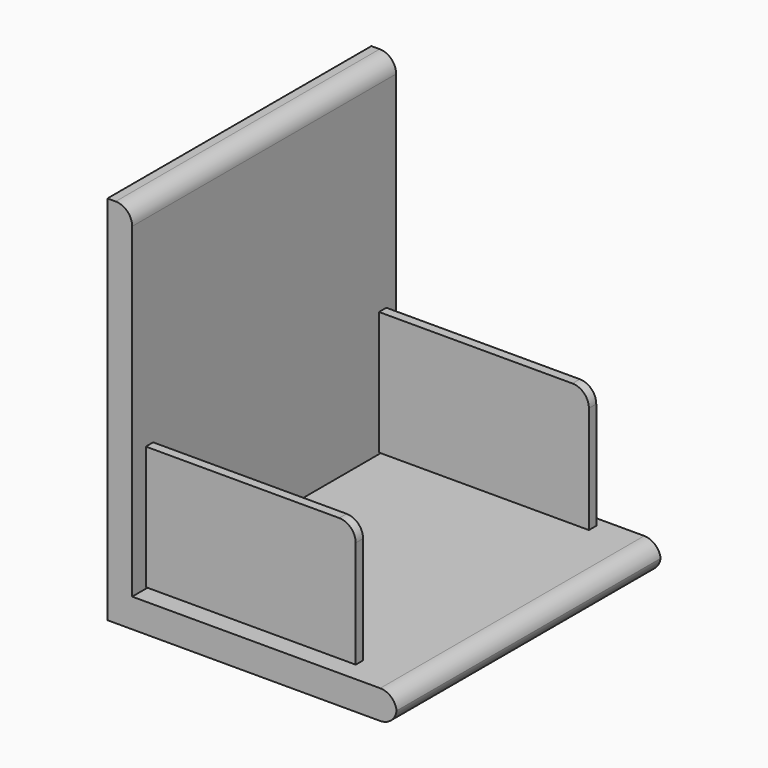
from build123d import *

# Parameters (mm, degrees)
F1_DEPTH      = 50.8
F2_W          = 64.6359566599
F2_H          = 2.8338059783
F3_DEPTH      = 38.1
F2_H_2        = 2.8299428523
F4_T1_DEPTH   = 127
F4_2_T1_DEPTH = 28.2338059783
F4_3_T1_DEPTH = 28.2299428523


# Not quite as in the source:
# - a fillet or chamfer that OpenCascade refuses, or shapes differently, is made with other operations: its cross-section is extruded or revolved along the edge and cut away or added


with BuildPart() as f1:
    # F0 (on Front) → F1 (new body, symmetric)
    with BuildSketch(Plane.XZ):
        Polygon((-46.0972779441, 66.8356441736), (-53.7172779441, 66.8356441736), (-53.7172779441, -47.4876239896), (-46.1948015571, -47.4876239896), (35.3699997067, -47.4876239896), (35.3699997067, -38.6183932424), (-46.0972779441, -38.6183932424), align=None)
    extrude(amount=F1_DEPTH, both=True)

    # F4: fillet of radius 5.08 on 3 edges, made by hand

    # F4_s2 → F4_t1 (cut)
    with BuildSketch(Plane.XZ.offset(-63.5)):
        with BuildLine():
            ThreePointArc((30.2899997067, -38.6183932424), (33.8821021552, -40.1062907939), (35.3699997067, -43.6983932424))
            Line((35.3699997067, -43.6983932424), (35.3699997067, -38.6183932424))
            Line((35.3699997067, -38.6183932424), (30.2899997067, -38.6183932424))
        make_face()
        with BuildLine():
            ThreePointArc((35.3699997067, -42.4076239896), (33.8821021552, -45.999726438), (30.2899997067, -47.4876239896))
            Line((30.2899997067, -47.4876239896), (35.3699997067, -47.4876239896))
            Line((35.3699997067, -47.4876239896), (35.3699997067, -42.4076239896))
        make_face()
        with BuildLine():
            ThreePointArc((-51.1772779441, 66.8356441736), (-47.5851754957, 65.347746622), (-46.0972779441, 61.7556441736))
            Line((-46.0972779441, 61.7556441736), (-46.0972779441, 66.8356441736))
            Line((-46.0972779441, 66.8356441736), (-51.1772779441, 66.8356441736))
        make_face()
    extrude(amount=F4_T1_DEPTH, mode=Mode.SUBTRACT)


with BuildPart() as f3:
    # F2 (on Top) → F3 (new body)
    with BuildSketch(Plane.XY):
        with Locations((-13.6866262183, 45.4956106842)):
            Rectangle(F2_W, F2_H)
    extrude(amount=-F3_DEPTH)

    # F4#2: fillet of radius 5.08 on 1 edges, made by hand

    # F4_2_s2 → F4_2_t1 (cut)
    with BuildSketch(Plane.XZ.offset(-59.6125136733)):
        with BuildLine():
            ThreePointArc((18.6313521117, -5.08), (17.1434545601, -1.4878975516), (13.5513521117, 0))
            Line((13.5513521117, 0), (18.6313521117, 0))
            Line((18.6313521117, 0), (18.6313521117, -5.08))
        make_face()
    extrude(amount=F4_2_T1_DEPTH, mode=Mode.SUBTRACT)


with BuildPart() as f3b:
    # F2 (on Top) → F3, piece 2 (new body)
    with BuildSketch(Plane.XY):
        with Locations((-13.6866262183, -44.2556086928)):
            Rectangle(F2_W, F2_H_2)
    extrude(amount=-F3_DEPTH)

    # F4#3: fillet of radius 5.08 on 1 edges, made by hand

    # F4_3_s2 → F4_3_t1 (cut)
    with BuildSketch(Plane.XZ.offset(30.1406372666)):
        with BuildLine():
            ThreePointArc((18.6313521117, -5.08), (17.1434545601, -1.4878975516), (13.5513521117, 0))
            Line((13.5513521117, 0), (18.6313521117, 0))
            Line((18.6313521117, 0), (18.6313521117, -5.08))
        make_face()
    extrude(amount=F4_3_T1_DEPTH, mode=Mode.SUBTRACT)


solid = Compound([f1.part, f3.part, f3b.part])
